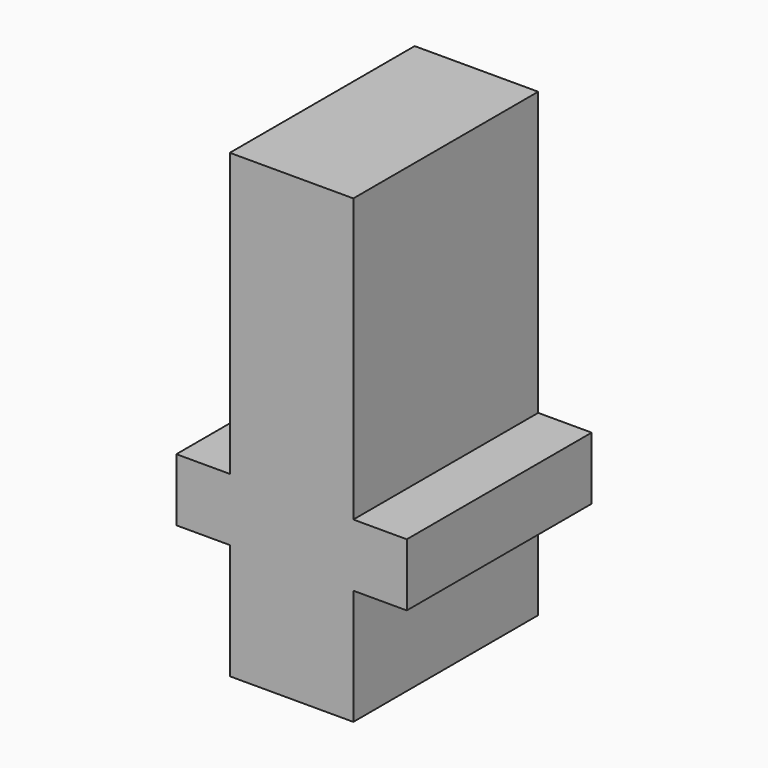
from build123d import *

# Parameters (mm, degrees)
F2_DEPTH = 4.7752


# Not quite as in the source:
# - a variable given as a bare number and used for a length is read in inches; the dataset says mm whatever the document's units were


with BuildPart() as f2:
    # F1 (on Front) → F2 (new body, symmetric)
    with BuildSketch(Plane.XZ):
        Polygon((-2.5527, 11.6857768009), (-2.5527, 0), (-4.7625, 0), (-4.7625, -2.5890231991), (-2.5527, -2.5890231991), (-2.5527, -7.3642231991), (2.5527, -7.3642231991), (2.5527, -2.5890231991), (4.7625, -2.5890231991), (4.7625, 0), (2.5527, 0), (2.5527, 11.6857768009), align=None)
    extrude(amount=F2_DEPTH, both=True)


solid = f2.part
